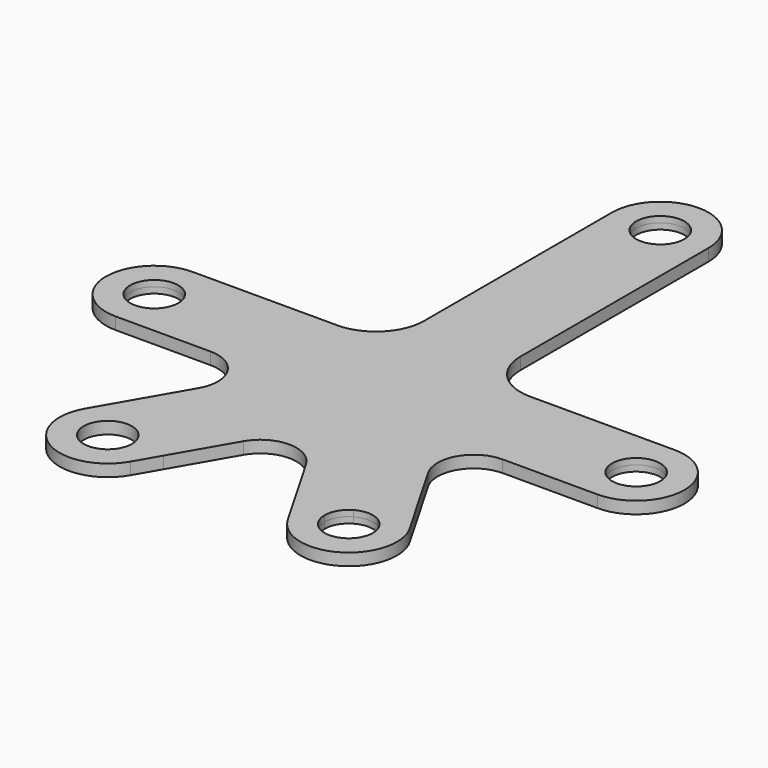
from build123d import *

# Parameters (mm, degrees)
F0_R     = 2
F1_DEPTH = 0.5


# Not quite as in the source:
# - a pattern or mirror of a feature is missing from the dataset's text; its kind, count and spacing are read off the source's solid


with BuildPart() as f1:
    # F0 (on Top) → F1 (new body)
    with BuildSketch(Plane.XY):
        with BuildLine():
            ThreePointArc((-20, 4), (-17.1715728753, 2.8284271247), (-16, 0))
            Line((-16, 0), (0, 0))
            Line((0, 0), (8, -13.8564064606))
            ThreePointArc((8, -13.8564064606), (10, -13.3205080757), (12, -13.8564064606))
            Line((12, -13.8564064606), (12.3094010768, -13.3205080757))
            Line((12.3094010768, -13.3205080757), (9.5262794416, -8.5))
            ThreePointArc((9.5262794416, -8.5), (9.5262794416, -5.5), (12.124355653, -4))
            Line((12.124355653, -4), (17.6905989232, -4))
            Line((17.6905989232, -4), (18, -3.4641016151))
            ThreePointArc((18, -3.4641016151), (16.1362966948, 1.0352761804), (20, 4))
            Line((20, 4), (8, 4))
            ThreePointArc((8, 4), (5.1715728753, 5.1715728753), (4, 8))
            Line((4, 8), (4, 27.5))
            ThreePointArc((4, 27.5), (0, 23.5), (-4, 27.5))
            Line((-4, 27.5), (-4, 8))
            ThreePointArc((-4, 8), (-5.1715728753, 5.1715728753), (-8, 4))
            Line((-8, 4), (-20, 4))
        make_face()
        with BuildLine():
            Line((0, 0), (-16, 0))
            ThreePointArc((-16, 0), (-16.5358983849, -2), (-18, -3.4641016151))
            Line((-18, -3.4641016151), (-17.6905989232, -4))
            Line((-17.6905989232, -4), (-12.124355653, -4))
            ThreePointArc((-12.124355653, -4), (-9.5262794416, -5.5), (-9.5262794416, -8.5))
            Line((-9.5262794416, -8.5), (-12.3094010768, -13.3205080757))
            Line((-12.3094010768, -13.3205080757), (-12, -13.8564064606))
            ThreePointArc((-12, -13.8564064606), (-10, -13.3205080757), (-8, -13.8564064606))
            Line((-8, -13.8564064606), (0, 0))
        make_face()
        with BuildLine():
            Line((8, -13.8564064606), (0, 0))
            Line((0, 0), (-8, -13.8564064606))
            ThreePointArc((-8, -13.8564064606), (-6.5358983849, -15.3205080757), (-6, -17.3205080757))
            Line((-6, -17.3205080757), (-5.3811978465, -17.3205080757))
            Line((-5.3811978465, -17.3205080757), (-2.5980762114, -12.5))
            ThreePointArc((-2.5980762114, -12.5), (0, -11), (2.5980762114, -12.5))
            Line((2.5980762114, -12.5), (5.3811978465, -17.3205080757))
            Line((5.3811978465, -17.3205080757), (6, -17.3205080757))
            ThreePointArc((6, -17.3205080757), (6.5358983849, -15.3205080757), (8, -13.8564064606))
        make_face()
        with BuildLine():
            Line((-9, -15.5884572681), (-8, -13.8564064606))
            ThreePointArc((-8, -13.8564064606), (-10, -13.3205080757), (-12, -13.8564064606))
            Line((-12, -13.8564064606), (-11, -15.5884572681))
            ThreePointArc((-11, -15.5884572681), (-10, -15.3205080757), (-9, -15.5884572681))
        make_face()
        with BuildLine():
            ThreePointArc((-6.5358983849, -19.3205080757), (-6.1362966948, -18.3557842561), (-6, -17.3205080757))
            Line((-6, -17.3205080757), (-8, -17.3205080757))
            ThreePointArc((-8, -17.3205080757), (-11, -19.0525588833), (-11, -15.5884572681))
            Line((-11, -15.5884572681), (-12, -13.8564064606))
            ThreePointArc((-12, -13.8564064606), (-12.8284271247, -14.4920809509), (-13.4641016151, -15.3205080757))
            ThreePointArc((-13.4641016151, -15.3205080757), (-12, -20.7846096908), (-6.5358983849, -19.3205080757))
        make_face()
        with BuildLine():
            ThreePointArc((-6, -17.3205080757), (-6.5358983849, -15.3205080757), (-8, -13.8564064606))
            Line((-8, -13.8564064606), (-9, -15.5884572681))
            ThreePointArc((-9, -15.5884572681), (-8.2679491924, -16.3205080757), (-8, -17.3205080757))
            Line((-8, -17.3205080757), (-6, -17.3205080757))
        make_face()
        with BuildLine():
            ThreePointArc((13.4641016151, -15.3205080757), (12.8284271247, -14.4920809509), (12, -13.8564064606))
            Line((12, -13.8564064606), (11, -15.5884572681))
            ThreePointArc((11, -15.5884572681), (11.7320508076, -16.3205080757), (12, -17.3205080757))
            ThreePointArc((12, -17.3205080757), (10, -19.3205080757), (8, -17.3205080757))
            Line((8, -17.3205080757), (6, -17.3205080757))
            ThreePointArc((6, -17.3205080757), (6.1362966948, -18.3557842561), (6.5358983849, -19.3205080757))
            ThreePointArc((6.5358983849, -19.3205080757), (11.0352761804, -21.1842113808), (14, -17.3205080757))
            ThreePointArc((14, -17.3205080757), (13.8637033052, -16.2852318953), (13.4641016151, -15.3205080757))
        make_face()
        with BuildLine():
            Line((9, -15.5884572681), (8, -13.8564064606))
            ThreePointArc((8, -13.8564064606), (6.5358983849, -15.3205080757), (6, -17.3205080757))
            Line((6, -17.3205080757), (8, -17.3205080757))
            ThreePointArc((8, -17.3205080757), (8.2679491924, -16.3205080757), (9, -15.5884572681))
        make_face()
        with BuildLine():
            ThreePointArc((12, -13.8564064606), (10, -13.3205080757), (8, -13.8564064606))
            Line((8, -13.8564064606), (9, -15.5884572681))
            ThreePointArc((9, -15.5884572681), (10, -15.3205080757), (11, -15.5884572681))
            Line((11, -15.5884572681), (12, -13.8564064606))
        make_face()
        with BuildLine():
            ThreePointArc((-19, -1.7320508076), (-21.7320508076, 1), (-18, 0))
            Line((-18, 0), (-16, 0))
            ThreePointArc((-16, 0), (-17.1715728753, 2.8284271247), (-20, 4))
            ThreePointArc((-20, 4), (-24, 0), (-20, -4))
            ThreePointArc((-20, -4), (-18.9647238196, -3.8637033052), (-18, -3.4641016151))
            Line((-18, -3.4641016151), (-19, -1.7320508076))
        make_face()
        with BuildLine():
            Line((-16, 0), (-18, 0))
            ThreePointArc((-18, 0), (-18.2679491924, -1), (-19, -1.7320508076))
            Line((-19, -1.7320508076), (-18, -3.4641016151))
            ThreePointArc((-18, -3.4641016151), (-16.5358983849, -2), (-16, 0))
        make_face()
        with BuildLine():
            ThreePointArc((20, 4), (16.1362966948, 1.0352761804), (18, -3.4641016151))
            ThreePointArc((18, -3.4641016151), (18.9647238196, -3.8637033052), (20, -4))
            ThreePointArc((20, -4), (22.8284271247, -2.8284271247), (24, 0))
            ThreePointArc((24, 0), (22.8284271247, 2.8284271247), (20, 4))
        make_face()
        with BuildLine():
            ThreePointArc((22, 0), (21, -1.7320508076), (19, -1.7320508076))
            ThreePointArc((19, -1.7320508076), (19, 1.7320508076), (22, 0))
        make_face(mode=Mode.SUBTRACT)
        with BuildLine():
            ThreePointArc((4, 27.5), (0, 31.5), (-4, 27.5))
            ThreePointArc((-4, 27.5), (0, 23.5), (4, 27.5))
        make_face()
        with Locations((0, 27.5)):
            Circle(F0_R, mode=Mode.SUBTRACT)
        with BuildLine():
            Line((-17.6905989232, -4), (-18, -3.4641016151))
            ThreePointArc((-18, -3.4641016151), (-18.9647238196, -3.8637033052), (-20, -4))
            Line((-20, -4), (-17.6905989232, -4))
        make_face()
        with BuildLine():
            Line((-12, -13.8564064606), (-12.3094010768, -13.3205080757))
            Line((-12.3094010768, -13.3205080757), (-13.4641016151, -15.3205080757))
            ThreePointArc((-13.4641016151, -15.3205080757), (-12.8284271247, -14.4920809509), (-12, -13.8564064606))
        make_face()
        with BuildLine():
            Line((-5.3811978465, -17.3205080757), (-6, -17.3205080757))
            ThreePointArc((-6, -17.3205080757), (-6.1362966948, -18.3557842561), (-6.5358983849, -19.3205080757))
            Line((-6.5358983849, -19.3205080757), (-5.3811978465, -17.3205080757))
        make_face()
        with BuildLine():
            ThreePointArc((6.5358983849, -19.3205080757), (6.1362966948, -18.3557842561), (6, -17.3205080757))
            Line((6, -17.3205080757), (5.3811978465, -17.3205080757))
            Line((5.3811978465, -17.3205080757), (6.5358983849, -19.3205080757))
        make_face()
        with BuildLine():
            Line((12.3094010768, -13.3205080757), (12, -13.8564064606))
            ThreePointArc((12, -13.8564064606), (12.8284271247, -14.4920809509), (13.4641016151, -15.3205080757))
            Line((13.4641016151, -15.3205080757), (12.3094010768, -13.3205080757))
        make_face()
        with BuildLine():
            Line((18, -3.4641016151), (17.6905989232, -4))
            Line((17.6905989232, -4), (20, -4))
            ThreePointArc((20, -4), (18.9647238196, -3.8637033052), (18, -3.4641016151))
        make_face()
    extrude(amount=F1_DEPTH)

    # F1_copies: F1 across plane


with BuildPart() as f1_1:
    add(f1.part)
    add(f1.part.mirror(Plane.XY.offset(0.5)))


solid = f1_1.part
